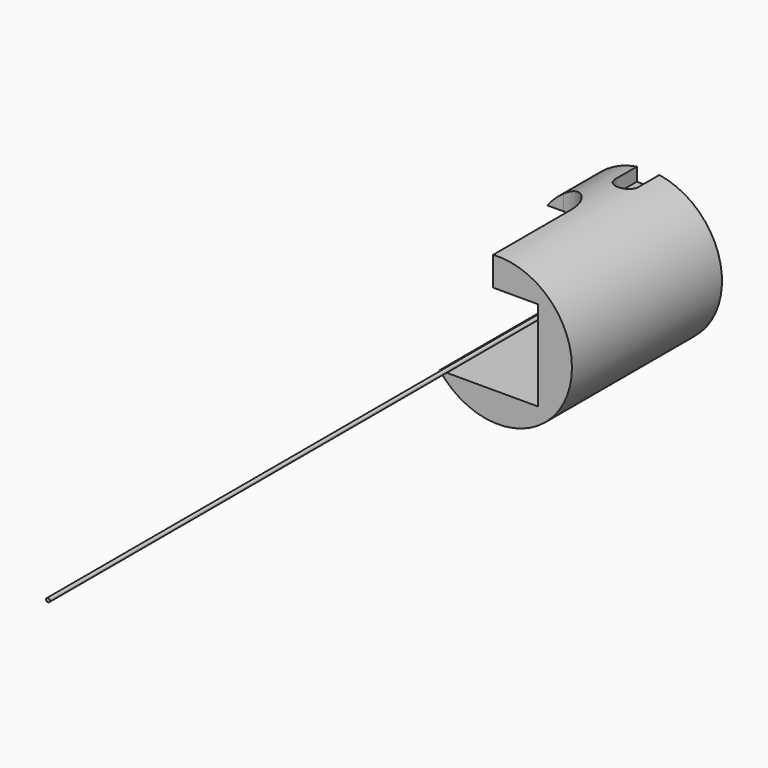
from build123d import *

# Parameters (mm, degrees)
F0_R      = 9.85
F1_DEPTH  = 25
F3_DEPTH  = 25
F5_DEPTH  = 5
F6_R      = 1.4999
F8_DEPTH  = 18
F9_R      = 5
F10_R     = 0.25
F11_DEPTH = 100


# Not quite as in the source:
# - a fillet or chamfer is up to 0.001 mm smaller than in the source, because OpenCascade refuses the exact size


with BuildPart() as f1:
    # F0 (on Front) → F1 (new body)
    with BuildSketch(Plane.XZ):
        Circle(F0_R)
    extrude(amount=-F1_DEPTH)

    # F2 (on face) → F3 (cut)
    with BuildSketch(Plane.XZ):
        with BuildLine():
            Line((5.2929249124, 5.9699154869), (-7.8347054239, 5.9699154869))
            ThreePointArc((-7.8347054239, 5.9699154869), (-9.8499269521, -0.0379346534), (-7.788490275, -6.0300845131))
            Line((-7.788490275, -6.0300845131), (5.2929249124, -6.0300845131))
            Line((5.2929249124, -6.0300845131), (5.2929249124, 5.9699154869))
        make_face()
    extrude(amount=-F3_DEPTH, mode=Mode.SUBTRACT)

    # F4 (on face) → F5 (cut)
    with BuildSketch(Plane(origin=(0, 25, 0), x_dir=(-1, 0, 0), z_dir=(0, 1, 0))):
        with BuildLine():
            ThreePointArc((1.5, 9.7351168457), (0, 9.85), (-1.5, 9.7351168457))
            Line((-1.5, 9.7351168457), (-1.5, 7.9699154869))
            Line((-1.5, 7.9699154869), (1.5, 7.9699154869))
            Line((1.5, 7.9699154869), (1.5, 9.7351168457))
        make_face()
    extrude(amount=-F5_DEPTH, mode=Mode.SUBTRACT)

    # F6 (radius 1.5 in the source; OpenCascade refuses exactly that, so slightly less here)
    f6_edges = [f1.edges().sort_by_distance(p)[0] for p in [
        (-1.5, 20, 8.852516),
        (1.5, 20, 8.852516),
    ]]
    fillet(f6_edges, radius=F6_R)

    # F7 (on face) → F8 (cut)
    with BuildSketch(Plane.XZ):
        with BuildLine():
            Line((-0.6592699745, 5.9699154869), (-0.6592699745, 9.8279124488))
            ThreePointArc((-0.6592699745, 9.8279124488), (-4.6645406694, 8.6755149901), (-7.8347054239, 5.9699154869))
            Line((-7.8347054239, 5.9699154869), (-0.6592699745, 5.9699154869))
        make_face()
    extrude(amount=-F8_DEPTH, mode=Mode.SUBTRACT)

    # F9
    f9_edges = [f1.edges().sort_by_distance(p)[0] for p in [
        (-0.65927, 18, 7.898914),
    ]]
    fillet(f9_edges, radius=F9_R)


with BuildPart() as f11:
    # F10 (on face) → F11 (new body)
    with BuildSketch(Plane(origin=(0, 25, 0), x_dir=(-1, 0, 0), z_dir=(0, 1, 0))):
        Circle(F10_R)
    extrude(amount=-F11_DEPTH)


solid = Compound([f1.part, f11.part])
